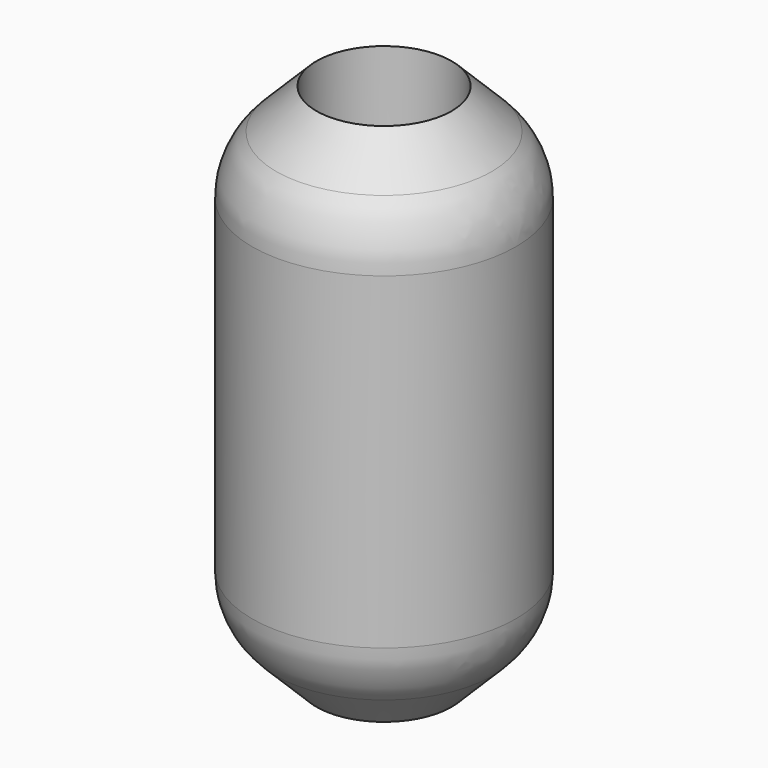
from build123d import *

# Parameters (mm, degrees)
F0_R     = 4.1
F0_R_2   = 3.5
F1_DEPTH = 0.5
F0_R_3   = 8
F2_DEPTH = 16
F5_R     = 5


# Not quite as in the source:
# - a fillet or chamfer that OpenCascade refuses, or shapes differently, is made with other operations: its cross-section is extruded or revolved along the edge and cut away or added


with BuildPart() as f1:
    # F0 (on Top) → F1 (new body, symmetric)
    with BuildSketch(Plane.XY):
        Circle(F0_R)
        Circle(F0_R_2, mode=Mode.SUBTRACT)
    extrude(amount=F1_DEPTH, both=True)

    # F0 (on Top) → F2 (join, symmetric)
    with BuildSketch(Plane.XY):
        Circle(F0_R_3)
        Circle(F0_R, mode=Mode.SUBTRACT)
    extrude(amount=F2_DEPTH, both=True)

    # F3: fillet of radius 1 on 2 edges, made by hand

    # F3_s1 → F3_t2 (revolve)
    with BuildSketch(Plane.XZ):
        with BuildLine():
            ThreePointArc((4.1, 1.416515139), (3.9366600265, 0.8687925815), (3.5, 0.5))
            Line((3.5, 0.5), (4.1, 0.5))
            Line((4.1, 0.5), (4.1, 1.416515139))
        make_face()
    revolve(axis=Axis((0, 0, 0.5), (0, 0, 1)))

    # F3_s3 → F3_t4 (revolve)
    with BuildSketch(Plane.XZ):
        with BuildLine():
            ThreePointArc((4.1, -1.416515139), (3.9366600265, -0.8687925815), (3.5, -0.5))
            Line((3.5, -0.5), (4.1, -0.5))
            Line((4.1, -0.5), (4.1, -1.416515139))
        make_face()
    revolve(axis=Axis((0, 0, -0.5), (0, 0, 1)))

    # F4: chamfer of 4 on 2 edges, made by hand

    # F4_s1 → F4_t2 (revolve, cut)
    with BuildSketch(Plane.XZ):
        Polygon((8, -12), (4, -16), (8, -16), align=None)
    revolve(axis=Axis((0, 0, -16), (0, 0, 1)), mode=Mode.SUBTRACT)

    # F4_s3 → F4_t4 (revolve, cut)
    with BuildSketch(Plane.XZ):
        Polygon((8, 12), (4, 16), (8, 16), align=None)
    revolve(axis=Axis((0, 0, 16), (0, 0, 1)), mode=Mode.SUBTRACT)

    # F5
    f5_edges = [f1.edges().sort_by_distance(p)[0] for p in [
        (-8, 0, -12),
        (-8, 0, 12),
    ]]
    fillet(f5_edges, radius=F5_R)


solid = f1.part
